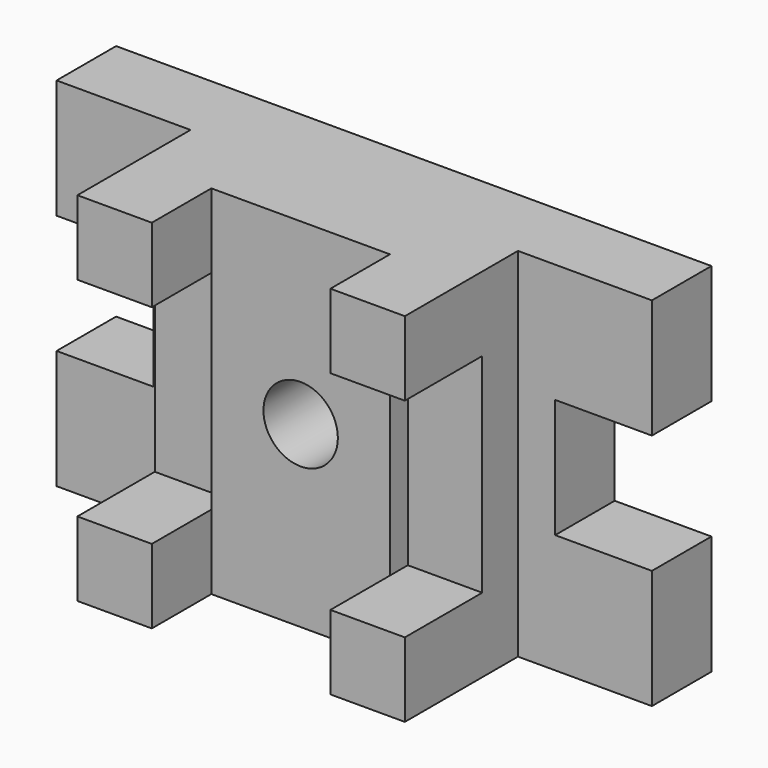
from build123d import *

# Parameters (mm, degrees)
F1_DEPTH = 15.875
F2_DEPTH = 46.0375
F0_R     = 7.9375
F3_DEPTH = 30.1625
F4_DEPTH = 25.4


with BuildPart() as f1:
    # F0 (on Front) → F1 (new body)
    with BuildSketch(Plane.XZ):
        Polygon((-28.1177360594, 50.8), (-56.6927360594, 50.8), (-56.6927360594, 25.4), (-36.0552360594, 25.4), (-36.0552360594, 0), (-56.6927360594, 0), (-56.6927360594, -25.4), (-28.1177360594, -25.4), (-28.1177360594, -9.525), (-28.1177360594, 34.925), align=None)
    extrude(amount=F1_DEPTH)

    # F0 (on Front) → F2 (join)
    with BuildSketch(Plane.XZ):
        Polygon((-12.2427360594, 50.8), (-28.1177360594, 50.8), (-28.1177360594, 34.925), (-20.1802360594, 34.925), (-12.2427360594, 34.925), align=None)
        Polygon((-20.1802360594, -9.525), (-28.1177360594, -9.525), (-28.1177360594, -25.4), (-12.2427360594, -25.4), (-12.2427360594, -9.525), align=None)
    extrude(amount=F2_DEPTH)



with BuildPart() as f1b:
    # F0 (on Front) → F1, piece 2 (new body)
    with BuildSketch(Plane.XZ):
        Polygon((70.3072639406, 50.8), (41.7322639406, 50.8), (41.7322639406, 34.925), (41.7322639406, -9.525), (41.7322639406, -25.4), (70.3072639406, -25.4), (70.3072639406, 0), (49.6697639406, 0), (49.6697639406, 25.4), (70.3072639406, 25.4), align=None)
    extrude(amount=F1_DEPTH)

    # F0 (on Front) → F2, piece 2 (join)
    with BuildSketch(Plane.XZ):
        Polygon((41.7322639406, 50.8), (25.8572639406, 50.8), (25.8572639406, 34.925), (33.7947639406, 34.925), (41.7322639406, 34.925), align=None)
        Polygon((33.7947639406, -9.525), (25.8572639406, -9.525), (25.8572639406, -25.4), (41.7322639406, -25.4), (41.7322639406, -9.525), align=None)
    extrude(amount=F2_DEPTH)


with BuildPart() as f1_1:
    add(f1.part)

    add(f1b.part)  # F3 merges F1b
    # F0 (on Front) → F3 (join)
    with BuildSketch(Plane.XZ):
        Polygon((25.8572639406, 50.8), (-12.2427360594, 50.8), (-12.2427360594, 34.925), (-12.2427360594, -9.525), (-12.2427360594, -25.4), (25.8572639406, -25.4), (25.8572639406, -9.525), (25.8572639406, 34.925), align=None)
        with Locations((6.8072639406, 12.7)):
            Circle(F0_R, mode=Mode.SUBTRACT)
    extrude(amount=F3_DEPTH)

    # F0 (on Front) → F4 (join)
    with BuildSketch(Plane.XZ):
        Polygon((-20.1802360594, 34.925), (-28.1177360594, 34.925), (-28.1177360594, -9.525), (-20.1802360594, -9.525), (-12.2427360594, -9.525), (-12.2427360594, 34.925), align=None)
        Polygon((33.7947639406, 34.925), (25.8572639406, 34.925), (25.8572639406, -9.525), (33.7947639406, -9.525), (41.7322639406, -9.525), (41.7322639406, 34.925), align=None)
    extrude(amount=F4_DEPTH)


solid = f1_1.part
